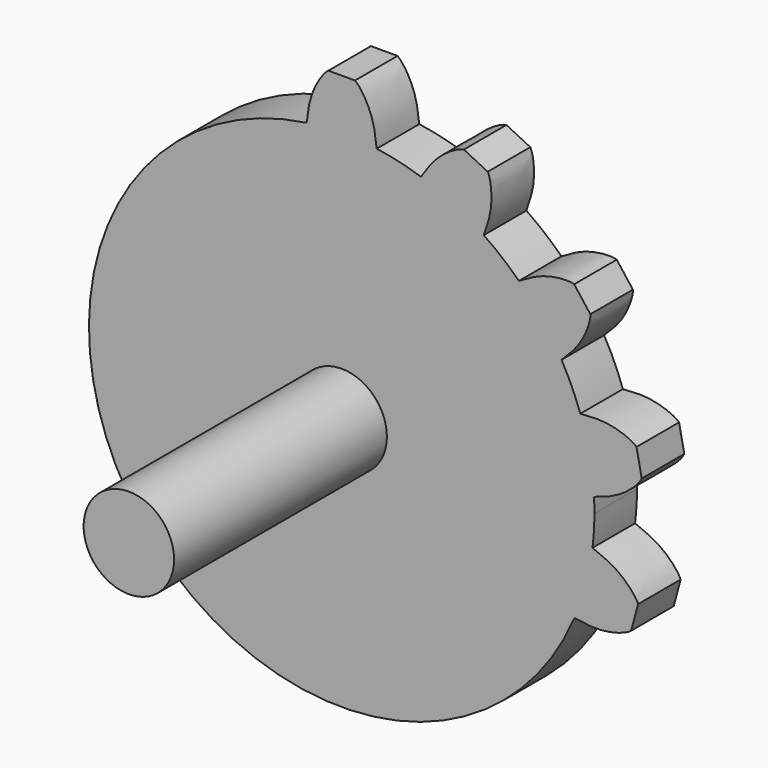
from build123d import *

# Parameters (mm, degrees)
F1_DEPTH        = 2.54
F2_DEPTH        = 2.54
F2_COPIES_COUNT = 5
F2_COPIES_ANGLE = 105
F3_R            = 2.159
F4_DEPTH        = 12.7


# Not quite as in the source:
# - a pattern or mirror of a feature is missing from the dataset's text; its kind, count and spacing are read off the source's solid


with BuildPart() as f1:
    # F0 (on Front) → F1 (new body)
    with BuildSketch(Plane.XZ):
        with BuildLine():
            ThreePointArc((-1.6725612742, 11.9485046673), (-7.917852399, -9.1033970795), (12.065, 0))
            ThreePointArc((12.065, 0), (9.1033970795, 7.917852399), (1.6725612742, 11.9485046673))
            ThreePointArc((1.6725612742, 11.9485046673), (0, 12.065), (-1.6725612742, 11.9485046673))
        make_face()
    extrude(amount=F1_DEPTH)

    # F0 (on Front) → F2 (join, through all)
    with BuildSketch(Plane.XZ):
        with BuildLine():
            ThreePointArc((-1.6725612742, 11.9485046673), (0, 12.065), (1.6725612742, 11.9485046673))
            add(Edge.make_bspline(
                [(1.6725612742, 11.9485046673), (1.6184790505, 12.4941120183), (1.4671756256, 13.4121286243), (0.8625889567, 14.3194638744), (0.635, 14.478)],
                knots=[0, 0, 0, 0, 0.5287892811, 1, 1, 1, 1], degree=3))
            Line((0.635, 14.478), (-0.635, 14.478))
            add(Edge.make_bspline(
                [(-1.6725612742, 11.9485046673), (-1.6184790505, 12.4941120183), (-1.4671756256, 13.4121286243), (-0.8625889567, 14.3194638744), (-0.635, 14.478)],
                knots=[0, 0, 0, 0, 0.5287892811, 1, 1, 1, 1], degree=3))
        make_face()
    f2 = extrude(amount=F2_DEPTH)

    # F2_copies: F2 ×5 about axis
    f2_copies_axis = Axis((0, 0, 0), (0, 1, 0))
    for i in range(1, F2_COPIES_COUNT):
        add(f2.rotate(f2_copies_axis, i * F2_COPIES_ANGLE / (F2_COPIES_COUNT - 1)))

    # F3 (on face) → F4 (join)
    with BuildSketch(Plane.XZ.offset(2.54)):
        Circle(F3_R)
    extrude(amount=F4_DEPTH)


solid = f1.part
